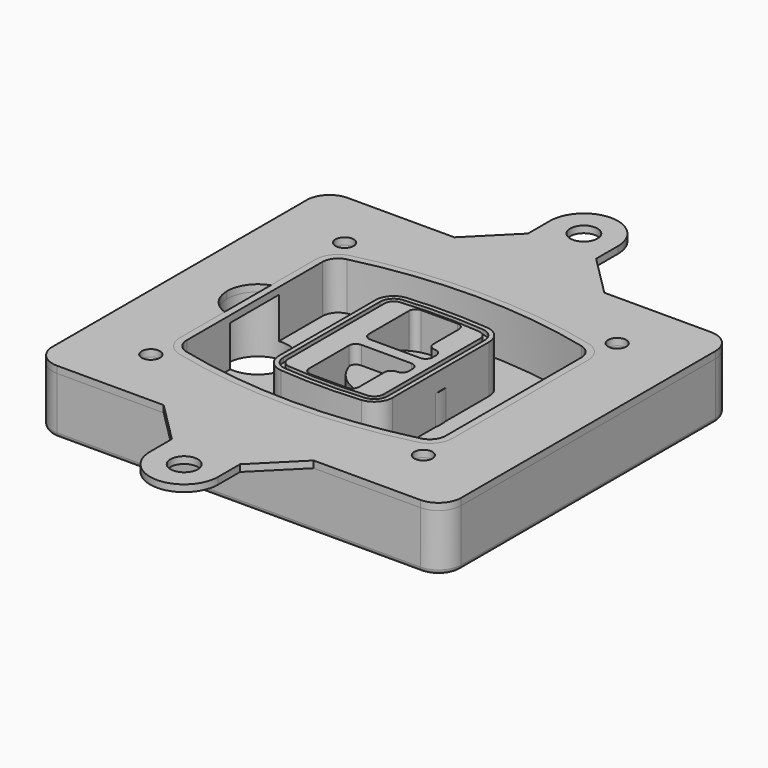
from build123d import *

# Parameters (mm, degrees)
F0_R      = 4
F1_DEPTH  = 25
F2_DEPTH  = 3
F3_DEPTH  = 18
F5_DEPTH  = 21
F6_DEPTH  = 2
F8_DEPTH  = 20
F9_DEPTH  = 16
F10_DEPTH = 25
F7_R      = 6
F7_R_2    = 4
F11_DEPTH = 6
F13_DEPTH = 9
F15_R     = 2
F16_R     = 6
F16_R_2   = 4
F17_DEPTH = 3


# Not quite as in the source:
# - a feature of the source that left no trace in its solid (it failed there, or was rolled back) is left out
# - a feature names something its author has since deleted; it is built from what else it names


with BuildPart() as f1:
    # F0 (on Top) → F1 (new body)
    with BuildSketch(Plane.XY):
        with BuildLine():
            ThreePointArc((-90, -70), (-87.0710678119, -77.0710678119), (-80, -80))
            Line((-80, -80), (80, -80))
            ThreePointArc((80, -80), (87.0710678119, -77.0710678119), (90, -70))
            Line((90, -70), (90, 70))
            ThreePointArc((90, 70), (87.0710678119, 77.0710678119), (80, 80))
            Line((80, 80), (-80, 80))
            ThreePointArc((-80, 80), (-87.0710678119, 77.0710678119), (-90, 70))
            Line((-90, 70), (-90, -70))
        make_face()
        with Locations((-60, -53.3333333333)):
            Circle(F0_R, mode=Mode.SUBTRACT)
        with Locations((60, -53.3333333333)):
            Circle(F0_R, mode=Mode.SUBTRACT)
        with Locations((-60, 53.3333333333)):
            Circle(F0_R, mode=Mode.SUBTRACT)
        with BuildLine():
            ThreePointArc((-64, 37.2990447398), (-61.0143011354, 45.9411029726), (-53.3306899286, 50.8970778549))
            ThreePointArc((-53.3306899286, 50.8970778549), (0, 57.3333333333), (53.3306899286, 50.8970778549))
            ThreePointArc((53.3306899286, 50.8970778549), (61.0143011354, 45.9411029726), (64, 37.2990447398))
            Line((64, 37.2990447398), (64, -37.2990447398))
            ThreePointArc((64, -37.2990447398), (61.0143011354, -45.9411029726), (53.3306899286, -50.8970778549))
            ThreePointArc((53.3306899286, -50.8970778549), (0, -57.3333333333), (-53.3306899286, -50.8970778549))
            ThreePointArc((-53.3306899286, -50.8970778549), (-61.0143011354, -45.9411029726), (-64, -37.2990447398))
            Line((-64, -37.2990447398), (-64, 37.2990447398))
        make_face(mode=Mode.SUBTRACT)
        with Locations((60, 53.3333333333)):
            Circle(F0_R, mode=Mode.SUBTRACT)
        with BuildLine():
            ThreePointArc((53.3306899286, 50.8970778549), (0, 57.3333333333), (-53.3306899286, 50.8970778549))
            ThreePointArc((-53.3306899286, 50.8970778549), (-61.0143011354, 45.9411029726), (-64, 37.2990447398))
            Line((-64, 37.2990447398), (-64, -37.2990447398))
            ThreePointArc((-64, -37.2990447398), (-61.0143011354, -45.9411029726), (-53.3306899286, -50.8970778549))
            ThreePointArc((-53.3306899286, -50.8970778549), (0, -57.3333333333), (53.3306899286, -50.8970778549))
            ThreePointArc((53.3306899286, -50.8970778549), (61.0143011354, -45.9411029726), (64, -37.2990447398))
            Line((64, -37.2990447398), (64, 37.2990447398))
            ThreePointArc((64, 37.2990447398), (61.0143011354, 45.9411029726), (53.3306899286, 50.8970778549))
        make_face()
        with BuildLine():
            Line((-60, -37.2990447398), (-60, 37.2990447398))
            ThreePointArc((-60, 37.2990447398), (-57.8673579538, 43.4719434775), (-52.3790642347, 47.0119255363))
            ThreePointArc((-52.3790642347, 47.0119255363), (0, 53.3333333333), (52.3790642347, 47.0119255363))
            ThreePointArc((52.3790642347, 47.0119255363), (57.8673579538, 43.4719434775), (60, 37.2990447398))
            Line((60, 37.2990447398), (60, -37.2990447398))
            ThreePointArc((60, -37.2990447398), (57.8673579538, -43.4719434775), (52.3790642347, -47.0119255363))
            ThreePointArc((52.3790642347, -47.0119255363), (0, -53.3333333333), (-52.3790642347, -47.0119255363))
            ThreePointArc((-52.3790642347, -47.0119255363), (-57.8673579538, -43.4719434775), (-60, -37.2990447398))
        make_face(mode=Mode.SUBTRACT)
        with BuildLine():
            ThreePointArc((-52.3790642347, 47.0119255363), (-57.8673579538, 43.4719434775), (-60, 37.2990447398))
            Line((-60, 37.2990447398), (-60, -37.2990447398))
            ThreePointArc((-60, -37.2990447398), (-57.8673579538, -43.4719434775), (-52.3790642347, -47.0119255363))
            ThreePointArc((-52.3790642347, -47.0119255363), (0, -53.3333333333), (52.3790642347, -47.0119255363))
            ThreePointArc((52.3790642347, -47.0119255363), (57.8673579538, -43.4719434775), (60, -37.2990447398))
            Line((60, -37.2990447398), (60, 37.2990447398))
            ThreePointArc((60, 37.2990447398), (57.8673579538, 43.4719434775), (52.3790642347, 47.0119255363))
            ThreePointArc((52.3790642347, 47.0119255363), (0, 53.3333333333), (-52.3790642347, 47.0119255363))
        make_face()
        with BuildLine():
            ThreePointArc((51.6653449643, 44.0980612973), (55.5071505677, 41.6200738562), (57, 37.2990447398))
            Line((57, 37.2990447398), (57, -37.2990447398))
            ThreePointArc((57, -37.2990447398), (55.5071505677, -41.6200738562), (51.6653449643, -44.0980612973))
            ThreePointArc((51.6653449643, -44.0980612973), (0, -50.3333333333), (-51.6653449643, -44.0980612973))
            ThreePointArc((-51.6653449643, -44.0980612973), (-55.5071505677, -41.6200738562), (-57, -37.2990447398))
            Line((-57, -37.2990447398), (-57, 37.2990447398))
            ThreePointArc((-57, 37.2990447398), (-55.5071505677, 41.6200738562), (-51.6653449643, 44.0980612973))
            ThreePointArc((-51.6653449643, 44.0980612973), (0, 50.3333333333), (51.6653449643, 44.0980612973))
        make_face(mode=Mode.SUBTRACT)
        with BuildLine():
            Line((57, -37.2990447398), (57, 37.2990447398))
            ThreePointArc((57, 37.2990447398), (55.5071505677, 41.6200738562), (51.6653449643, 44.0980612973))
            ThreePointArc((51.6653449643, 44.0980612973), (0, 50.3333333333), (-51.6653449643, 44.0980612973))
            ThreePointArc((-51.6653449643, 44.0980612973), (-55.5071505677, 41.6200738562), (-57, 37.2990447398))
            Line((-57, 37.2990447398), (-57, -37.2990447398))
            ThreePointArc((-57, -37.2990447398), (-55.5071505677, -41.6200738562), (-51.6653449643, -44.0980612973))
            ThreePointArc((-51.6653449643, -44.0980612973), (0, -50.3333333333), (51.6653449643, -44.0980612973))
            ThreePointArc((51.6653449643, -44.0980612973), (55.5071505677, -41.6200738562), (57, -37.2990447398))
        make_face()
    extrude(amount=-F1_DEPTH)

    # F0 (on Top) → F2 (join)
    with BuildSketch(Plane.XY):
        with BuildLine():
            ThreePointArc((-52.3790642347, 47.0119255363), (-57.8673579538, 43.4719434775), (-60, 37.2990447398))
            Line((-60, 37.2990447398), (-60, -37.2990447398))
            ThreePointArc((-60, -37.2990447398), (-57.8673579538, -43.4719434775), (-52.3790642347, -47.0119255363))
            ThreePointArc((-52.3790642347, -47.0119255363), (0, -53.3333333333), (52.3790642347, -47.0119255363))
            ThreePointArc((52.3790642347, -47.0119255363), (57.8673579538, -43.4719434775), (60, -37.2990447398))
            Line((60, -37.2990447398), (60, 37.2990447398))
            ThreePointArc((60, 37.2990447398), (57.8673579538, 43.4719434775), (52.3790642347, 47.0119255363))
            ThreePointArc((52.3790642347, 47.0119255363), (0, 53.3333333333), (-52.3790642347, 47.0119255363))
        make_face()
        with BuildLine():
            ThreePointArc((51.6653449643, 44.0980612973), (55.5071505677, 41.6200738562), (57, 37.2990447398))
            Line((57, 37.2990447398), (57, -37.2990447398))
            ThreePointArc((57, -37.2990447398), (55.5071505677, -41.6200738562), (51.6653449643, -44.0980612973))
            ThreePointArc((51.6653449643, -44.0980612973), (0, -50.3333333333), (-51.6653449643, -44.0980612973))
            ThreePointArc((-51.6653449643, -44.0980612973), (-55.5071505677, -41.6200738562), (-57, -37.2990447398))
            Line((-57, -37.2990447398), (-57, 37.2990447398))
            ThreePointArc((-57, 37.2990447398), (-55.5071505677, 41.6200738562), (-51.6653449643, 44.0980612973))
            ThreePointArc((-51.6653449643, 44.0980612973), (0, 50.3333333333), (51.6653449643, 44.0980612973))
        make_face(mode=Mode.SUBTRACT)
    extrude(amount=F2_DEPTH)

    # F0 (on Top) → F3 (cut)
    with BuildSketch(Plane.XY):
        with BuildLine():
            Line((57, -37.2990447398), (57, 37.2990447398))
            ThreePointArc((57, 37.2990447398), (55.5071505677, 41.6200738562), (51.6653449643, 44.0980612973))
            ThreePointArc((51.6653449643, 44.0980612973), (0, 50.3333333333), (-51.6653449643, 44.0980612973))
            ThreePointArc((-51.6653449643, 44.0980612973), (-55.5071505677, 41.6200738562), (-57, 37.2990447398))
            Line((-57, 37.2990447398), (-57, -37.2990447398))
            ThreePointArc((-57, -37.2990447398), (-55.5071505677, -41.6200738562), (-51.6653449643, -44.0980612973))
            ThreePointArc((-51.6653449643, -44.0980612973), (0, -50.3333333333), (51.6653449643, -44.0980612973))
            ThreePointArc((51.6653449643, -44.0980612973), (55.5071505677, -41.6200738562), (57, -37.2990447398))
        make_face()
    extrude(amount=-F3_DEPTH, mode=Mode.SUBTRACT)

    # F4 (on face) → F5 (join, through all)
    with BuildSketch(Plane.XY.offset(3)):
        with BuildLine():
            ThreePointArc((-25, -26.587695628), (-22.8992979869, -31.9912392117), (-17.7004291845, -34.5569740744))
            ThreePointArc((-17.7004291845, -34.5569740744), (0, -35.3333333333), (17.7004291845, -34.5569740744))
            ThreePointArc((17.7004291845, -34.5569740744), (22.8992979869, -31.9912392117), (25, -26.587695628))
            Line((25, -26.587695628), (25, 26.587695628))
            ThreePointArc((25, 26.587695628), (22.8992979869, 31.9912392117), (17.7004291845, 34.5569740744))
            ThreePointArc((17.7004291845, 34.5569740744), (0, 35.3333333333), (-17.7004291845, 34.5569740744))
            ThreePointArc((-17.7004291845, 34.5569740744), (-22.8992979869, 31.9912392117), (-25, 26.587695628))
            Line((-25, 26.587695628), (-25, -26.587695628))
        make_face()
        with BuildLine():
            ThreePointArc((17.5253218884, 32.5646544628), (21.4244734902, 30.6403533158), (23, 26.587695628))
            Line((23, 26.587695628), (23, -26.587695628))
            ThreePointArc((23, -26.587695628), (21.4244734902, -30.6403533158), (17.5253218884, -32.5646544628))
            ThreePointArc((17.5253218884, -32.5646544628), (0, -33.3333333333), (-17.5253218884, -32.5646544628))
            ThreePointArc((-17.5253218884, -32.5646544628), (-21.4244734902, -30.6403533158), (-23, -26.587695628))
            Line((-23, -26.587695628), (-23, 26.587695628))
            ThreePointArc((-23, 26.587695628), (-21.4244734902, 30.6403533158), (-17.5253218884, 32.5646544628))
            ThreePointArc((-17.5253218884, 32.5646544628), (0, 33.3333333333), (17.5253218884, 32.5646544628))
        make_face(mode=Mode.SUBTRACT)
        with BuildLine():
            Line((23, -26.587695628), (23, 26.587695628))
            ThreePointArc((23, 26.587695628), (21.4244734902, 30.6403533158), (17.5253218884, 32.5646544628))
            ThreePointArc((17.5253218884, 32.5646544628), (0, 33.3333333333), (-17.5253218884, 32.5646544628))
            ThreePointArc((-17.5253218884, 32.5646544628), (-21.4244734902, 30.6403533158), (-23, 26.587695628))
            Line((-23, 26.587695628), (-23, -26.587695628))
            ThreePointArc((-23, -26.587695628), (-21.4244734902, -30.6403533158), (-17.5253218884, -32.5646544628))
            ThreePointArc((-17.5253218884, -32.5646544628), (0, -33.3333333333), (17.5253218884, -32.5646544628))
            ThreePointArc((17.5253218884, -32.5646544628), (21.4244734902, -30.6403533158), (23, -26.587695628))
        make_face()
        with BuildLine():
            ThreePointArc((17.3502145923, 30.5723348512), (19.9496489934, 29.2894674198), (21, 26.587695628))
            Line((21, 26.587695628), (21, -26.587695628))
            ThreePointArc((21, -26.587695628), (19.9496489934, -29.2894674198), (17.3502145923, -30.5723348512))
            ThreePointArc((17.3502145923, -30.5723348512), (0, -31.3333333333), (-17.3502145923, -30.5723348512))
            ThreePointArc((-17.3502145923, -30.5723348512), (-19.9496489934, -29.2894674198), (-21, -26.587695628))
            Line((-21, -26.587695628), (-21, 26.587695628))
            ThreePointArc((-21, 26.587695628), (-19.9496489934, 29.2894674198), (-17.3502145923, 30.5723348512))
            ThreePointArc((-17.3502145923, 30.5723348512), (0, 31.3333333333), (17.3502145923, 30.5723348512))
        make_face(mode=Mode.SUBTRACT)
        with BuildLine():
            Line((21, -26.587695628), (21, 26.587695628))
            ThreePointArc((21, 26.587695628), (19.9496489934, 29.2894674198), (17.3502145923, 30.5723348512))
            ThreePointArc((17.3502145923, 30.5723348512), (0, 31.3333333333), (-17.3502145923, 30.5723348512))
            ThreePointArc((-17.3502145923, 30.5723348512), (-19.9496489934, 29.2894674198), (-21, 26.587695628))
            Line((-21, 26.587695628), (-21, -26.587695628))
            ThreePointArc((-21, -26.587695628), (-19.9496489934, -29.2894674198), (-17.3502145923, -30.5723348512))
            ThreePointArc((-17.3502145923, -30.5723348512), (0, -31.3333333333), (17.3502145923, -30.5723348512))
            ThreePointArc((17.3502145923, -30.5723348512), (19.9496489934, -29.2894674198), (21, -26.587695628))
        make_face()
        with BuildLine():
            Line((-8, -2.5), (14, -2.5))
            ThreePointArc((14, -2.5), (16.1213203436, -3.3786796564), (17, -5.5))
            Line((17, -5.5), (17, -7.5))
            ThreePointArc((17, -7.5), (16.1213203436, -9.6213203436), (14, -10.5))
            ThreePointArc((14, -10.5), (11.8786796564, -11.3786796564), (11, -13.5))
            Line((11, -13.5), (11, -27.5))
            ThreePointArc((11, -27.5), (10.1213203436, -29.6213203436), (8, -30.5))
            Line((8, -30.5), (-8, -30.5))
            ThreePointArc((-8, -30.5), (-10.1213203436, -29.6213203436), (-11, -27.5))
            Line((-11, -27.5), (-11, -5.5))
            ThreePointArc((-11, -5.5), (-10.1213203436, -3.3786796564), (-8, -2.5))
        make_face(mode=Mode.SUBTRACT)
        with BuildLine():
            ThreePointArc((-8, 2.5), (-10.1213203436, 3.3786796564), (-11, 5.5))
            Line((-11, 5.5), (-11, 27.5))
            ThreePointArc((-11, 27.5), (-10.1213203436, 29.6213203436), (-8, 30.5))
            Line((-8, 30.5), (8, 30.5))
            ThreePointArc((8, 30.5), (10.1213203436, 29.6213203436), (11, 27.5))
            Line((11, 27.5), (11, 13.5))
            ThreePointArc((11, 13.5), (11.8786796564, 11.3786796564), (14, 10.5))
            ThreePointArc((14, 10.5), (16.1213203436, 9.6213203436), (17, 7.5))
            Line((17, 7.5), (17, 5.5))
            ThreePointArc((17, 5.5), (16.1213203436, 3.3786796564), (14, 2.5))
            Line((14, 2.5), (-8, 2.5))
        make_face(mode=Mode.SUBTRACT)
    extrude(amount=-F5_DEPTH)

    # F4 (on face) → F6 (cut)
    with BuildSketch(Plane.XY.offset(3)):
        with BuildLine():
            Line((23, -26.587695628), (23, 26.587695628))
            ThreePointArc((23, 26.587695628), (21.4244734902, 30.6403533158), (17.5253218884, 32.5646544628))
            ThreePointArc((17.5253218884, 32.5646544628), (0, 33.3333333333), (-17.5253218884, 32.5646544628))
            ThreePointArc((-17.5253218884, 32.5646544628), (-21.4244734902, 30.6403533158), (-23, 26.587695628))
            Line((-23, 26.587695628), (-23, -26.587695628))
            ThreePointArc((-23, -26.587695628), (-21.4244734902, -30.6403533158), (-17.5253218884, -32.5646544628))
            ThreePointArc((-17.5253218884, -32.5646544628), (0, -33.3333333333), (17.5253218884, -32.5646544628))
            ThreePointArc((17.5253218884, -32.5646544628), (21.4244734902, -30.6403533158), (23, -26.587695628))
        make_face()
        with BuildLine():
            ThreePointArc((17.3502145923, 30.5723348512), (19.9496489934, 29.2894674198), (21, 26.587695628))
            Line((21, 26.587695628), (21, -26.587695628))
            ThreePointArc((21, -26.587695628), (19.9496489934, -29.2894674198), (17.3502145923, -30.5723348512))
            ThreePointArc((17.3502145923, -30.5723348512), (0, -31.3333333333), (-17.3502145923, -30.5723348512))
            ThreePointArc((-17.3502145923, -30.5723348512), (-19.9496489934, -29.2894674198), (-21, -26.587695628))
            Line((-21, -26.587695628), (-21, 26.587695628))
            ThreePointArc((-21, 26.587695628), (-19.9496489934, 29.2894674198), (-17.3502145923, 30.5723348512))
            ThreePointArc((-17.3502145923, 30.5723348512), (0, 31.3333333333), (17.3502145923, 30.5723348512))
        make_face(mode=Mode.SUBTRACT)
    extrude(amount=-F6_DEPTH, mode=Mode.SUBTRACT)

    # F7 (on face) → F8 (join)
    with BuildSketch(Plane(origin=(0, 0, -25), x_dir=(1, 0, 0), z_dir=(0, 0, -1))):
        with BuildLine():
            ThreePointArc((-6.71157564, 0), (6.7567035675, 13.4682792075), (20.224982775, 0))
            Line((20.224982775, 0), (25.224982775, 0))
            ThreePointArc((25.224982775, 0), (6.7567035675, 18.4682792075), (-11.71157564, 0))
            Line((-11.71157564, 0), (-6.71157564, 0))
        make_face()
        with BuildLine():
            Line((-6.71157564, 0), (20.224982775, 0))
            ThreePointArc((20.224982775, 0), (6.7567035675, 13.4682792075), (-6.71157564, 0))
        make_face()
        with BuildLine():
            ThreePointArc((-6.71157564, 0), (6.7567035675, -13.4682792075), (20.224982775, 0))
            Line((20.224982775, 0), (-6.71157564, 0))
        make_face()
        with BuildLine():
            Line((25.224982775, 0), (20.224982775, 0))
            ThreePointArc((20.224982775, 0), (6.7567035675, -13.4682792075), (-6.71157564, 0))
            Line((-6.71157564, 0), (-11.71157564, 0))
            ThreePointArc((-11.71157564, 0), (6.7567035675, -18.4682792075), (25.224982775, 0))
        make_face()
    extrude(amount=-F8_DEPTH)

    # F7 (on face) → F9 (cut)
    with BuildSketch(Plane(origin=(0, 0, -25), x_dir=(1, 0, 0), z_dir=(0, 0, -1))):
        with BuildLine():
            Line((-6.71157564, 0), (20.224982775, 0))
            ThreePointArc((20.224982775, 0), (6.7567035675, 13.4682792075), (-6.71157564, 0))
        make_face()
        with BuildLine():
            ThreePointArc((-6.71157564, 0), (6.7567035675, -13.4682792075), (20.224982775, 0))
            Line((20.224982775, 0), (-6.71157564, 0))
        make_face()
    extrude(amount=-F9_DEPTH, mode=Mode.SUBTRACT)

    # F7 (on face) → F10 (cut)
    with BuildSketch(Plane(origin=(0, 0, -25), x_dir=(1, 0, 0), z_dir=(0, 0, -1))):
        with BuildLine():
            Line((-69.0318229325, 0), (-42.0952645175, 0))
            ThreePointArc((-42.0952645175, 0), (-55.563543725, 13.4682792075), (-69.0318229325, 0))
        make_face()
        with BuildLine():
            ThreePointArc((-69.0318229325, 0), (-55.563543725, -13.4682792075), (-42.0952645175, 0))
            Line((-42.0952645175, 0), (-69.0318229325, 0))
        make_face()
    extrude(amount=-F10_DEPTH, mode=Mode.SUBTRACT)

    # F7 (on face) → F11 (cut)
    with BuildSketch(Plane(origin=(0, 0, -25), x_dir=(1, 0, 0), z_dir=(0, 0, -1))):
        with Locations((60, -53.3333333333)):
            Circle(F7_R)
        with Locations((60, -53.3333333333)):
            Circle(F7_R_2, mode=Mode.SUBTRACT)
        with Locations((-60, -53.3333333333)):
            Circle(F7_R)
        with Locations((-60, -53.3333333333)):
            Circle(F7_R_2, mode=Mode.SUBTRACT)
        with Locations((-60, 53.3333333333)):
            Circle(F7_R)
        with Locations((-60, 53.3333333333)):
            Circle(F7_R_2, mode=Mode.SUBTRACT)
        with Locations((60, 53.3333333333)):
            Circle(F7_R)
        with Locations((60, 53.3333333333)):
            Circle(F7_R_2, mode=Mode.SUBTRACT)
    extrude(amount=-F11_DEPTH, mode=Mode.SUBTRACT)

    # F12 (on face) → F13 (cut, through all)
    with BuildSketch(Plane(origin=(0, 0, -9), x_dir=(1, 0, 0), z_dir=(0, 0, -1))):
        with BuildLine():
            ThreePointArc((20.224982775, 0), (20.1663399806, 1.2554664788), (19.9909222755, 2.5))
            Line((19.9909222755, 2.5), (14, 2.5))
            ThreePointArc((14, 2.5), (16.1213203436, 3.3786796564), (17, 5.5))
            Line((17, 5.5), (17, 7.5))
            ThreePointArc((17, 7.5), (16.1213203436, 9.6213203436), (14, 10.5))
            ThreePointArc((14, 10.5), (12.1627255951, 11.1284134507), (11.0951631559, 12.750384826))
            ThreePointArc((11.0951631559, 12.750384826), (11.0476113807, 12.7664660322), (11, 12.7823698976))
            Line((11, 12.7823698976), (11, -12.7823698976))
            ThreePointArc((11, -12.7823698976), (11.0476113807, -12.7664660322), (11.0951631559, -12.750384826))
            ThreePointArc((11.0951631559, -12.750384826), (12.1627255951, -11.1284134507), (14, -10.5))
            ThreePointArc((14, -10.5), (16.1213203436, -9.6213203436), (17, -7.5))
            Line((17, -7.5), (17, -5.5))
            ThreePointArc((17, -5.5), (16.1213203436, -3.3786796564), (14, -2.5))
            Line((14, -2.5), (19.9909222755, -2.5))
            ThreePointArc((19.9909222755, -2.5), (20.1663399806, -1.2554664788), (20.224982775, 0))
        make_face()
    extrude(amount=F13_DEPTH, mode=Mode.SUBTRACT)

    # F15
    f15_edges = [f1.edges().sort_by_distance(p)[0] for p in [
        (0, -80, -25),
        (-87.071068, -77.071068, -25),
        (-90, 0, -25),
        (-87.071068, 77.071068, -25),
        (87.071068, -77.071068, -25),
        (0, 80, -25),
        (90, 0, -25),
        (87.071068, 77.071068, -25),
    ]]
    fillet(f15_edges, radius=F15_R)


with BuildPart() as f17:
    # F16 (on face) → F17 (new body, through all)
    with BuildSketch(Plane.XY):
        with BuildLine():
            Line((15, 98), (15, 110))
            ThreePointArc((15, 110), (0, 125), (-15, 110))
            Line((-15, 110), (-15, 98))
            Line((-15, 98), (-33, 80))
            Line((-33, 80), (33, 80))
            Line((33, 80), (15, 98))
        make_face()
        with Locations((0, 110)):
            Circle(F16_R, mode=Mode.SUBTRACT)
        with BuildLine():
            Line((15, -98), (33, -80))
            Line((33, -80), (-33, -80))
            Line((-33, -80), (-15, -98))
            Line((-15, -98), (-15, -110))
            ThreePointArc((-15, -110), (0, -125), (15, -110))
            Line((15, -110), (15, -98))
        make_face()
        with Locations((0, -110)):
            Circle(F16_R, mode=Mode.SUBTRACT)
        with BuildLine():
            Line((80, 80), (33, 80))
            Line((33, 80), (-33, 80))
            Line((-33, 80), (-80, 80))
            ThreePointArc((-80, 80), (-87.0710678119, 77.0710678119), (-90, 70))
            Line((-90, 70), (-90, -70))
            ThreePointArc((-90, -70), (-87.0710678119, -77.0710678119), (-80, -80))
            Line((-80, -80), (-33, -80))
            Line((-33, -80), (33, -80))
            Line((33, -80), (80, -80))
            ThreePointArc((80, -80), (87.0710678119, -77.0710678119), (90, -70))
            Line((90, -70), (90, 70))
            ThreePointArc((90, 70), (87.0710678119, 77.0710678119), (80, 80))
        make_face()
        with Locations((-60, -53.3333333333)):
            Circle(F16_R_2, mode=Mode.SUBTRACT)
        with BuildLine():
            ThreePointArc((-60, 37.2990447398), (-57.8673579538, 43.4719434775), (-52.3790642347, 47.0119255363))
            ThreePointArc((-52.3790642347, 47.0119255363), (0, 53.3333333333), (52.3790642347, 47.0119255363))
            ThreePointArc((52.3790642347, 47.0119255363), (57.8673579538, 43.4719434775), (60, 37.2990447398))
            Line((60, 37.2990447398), (60, -37.2990447398))
            ThreePointArc((60, -37.2990447398), (57.8673579538, -43.4719434775), (52.3790642347, -47.0119255363))
            ThreePointArc((52.3790642347, -47.0119255363), (0, -53.3333333333), (-52.3790642347, -47.0119255363))
            ThreePointArc((-52.3790642347, -47.0119255363), (-57.8673579538, -43.4719434775), (-60, -37.2990447398))
            Line((-60, -37.2990447398), (-60, -12.7166190685))
            ThreePointArc((-60, -12.7166190685), (-66.5441169481, -7.798817635), (-69.0318229325, 0))
            ThreePointArc((-69.0318229325, 0), (-66.5441169481, 7.798817635), (-60, 12.7166190685))
            Line((-60, 12.7166190685), (-60, 37.2990447398))
        make_face(mode=Mode.SUBTRACT)
        with Locations((60, -53.3333333333)):
            Circle(F16_R_2, mode=Mode.SUBTRACT)
        with Locations((-60, 53.3333333333)):
            Circle(F16_R_2, mode=Mode.SUBTRACT)
        with Locations((60, 53.3333333333)):
            Circle(F16_R_2, mode=Mode.SUBTRACT)
    extrude(amount=F17_DEPTH)


solid = Compound([f1.part, f17.part])
